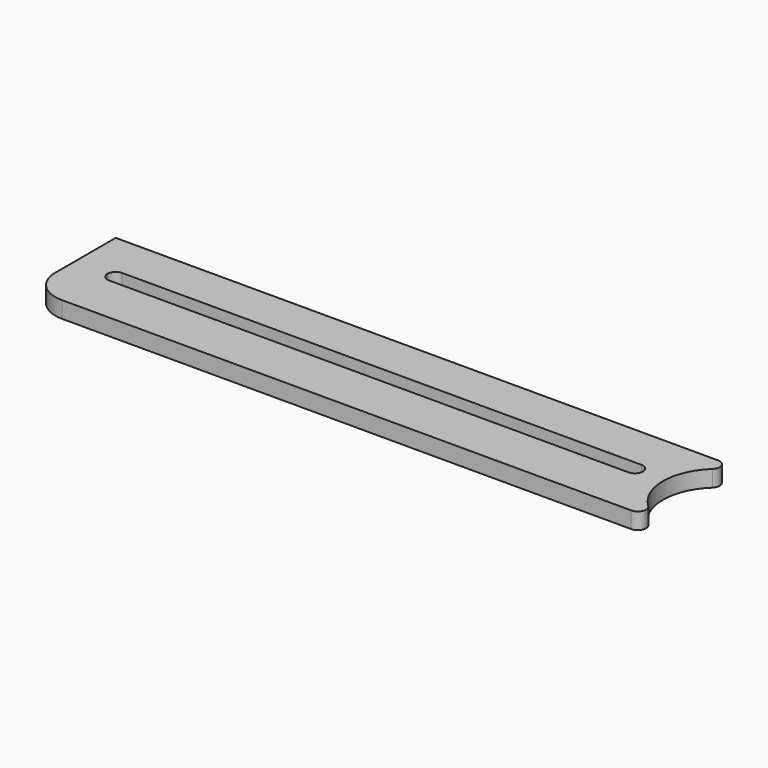
from build123d import *

# Parameters (mm, degrees)
F0_W         = 99.7252352536
F0_H         = 16.7486164719
F1_DEPTH     = 2.54
F2_R         = 5.08
F3_R         = 8.5048235264
F4_DEPTH     = 2.54
F5_W         = 82.7053110433
F5_H         = 2.5119255297
F6_DEPTH     = 2.54
F7_R         = 1.27
F8_T1_DEPTH  = 2.54
F9_R         = 1.27
F10_T1_DEPTH = 2.54
F11_R        = 1.27
F12_R        = 1.27


# Not quite as in the source:
# - a fillet or chamfer that OpenCascade refuses, or shapes differently, is made with other operations: its cross-section is extruded or revolved along the edge and cut away or added


with BuildPart() as f1:
    # F0 (on Top) → F1 (new body)
    with BuildSketch(Plane.XY):
        with Locations((-11.1071113497, -8.3743082359)):
            Rectangle(F0_W, F0_H)
    extrude(amount=F1_DEPTH)

    # F2
    f2_edges = [f1.edges().sort_by_distance(p)[0] for p in [
        (-60.969729, -16.748616, 1.27),
    ]]
    fillet(f2_edges, radius=F2_R)

    # F3 (on face) → F4 (cut)
    with BuildSketch(Plane.XY.offset(2.54)):
        with Locations((38.7555062771, -8.3743082359)):
            Circle(F3_R)
    extrude(amount=-F4_DEPTH, mode=Mode.SUBTRACT)

    # F5 (on face) → F6 (cut)
    with BuildSketch(Plane(origin=(0, 0, 0), x_dir=(1, 0, 0), z_dir=(0, 0, -1))):
        with Locations((-14.5370734549, 7.9348592553)):
            Rectangle(F5_W, F5_H)
    extrude(amount=-F6_DEPTH, mode=Mode.SUBTRACT)

    # F7
    f7_edges = [f1.edges().sort_by_distance(p)[0] for p in [
        (-55.889729, -9.190822, 1.27),
    ]]
    fillet(f7_edges, radius=F7_R)

    # F8: fillet of radius 1.27 on 1 edges, made by hand

    # F8_s2 → F8_t1 (join)
    with BuildSketch(Plane.XY):
        with BuildLine():
            ThreePointArc((-55.8897289765, -7.9488964905), (-55.5177545886, -7.0508708784), (-54.6197289765, -6.6788964905))
            Line((-54.6197289765, -6.6788964905), (-55.8897289765, -6.6788964905))
            Line((-55.8897289765, -6.6788964905), (-55.8897289765, -7.9488964905))
        make_face()
    extrude(amount=F8_T1_DEPTH)

    # F9
    f9_edges = [f1.edges().sort_by_distance(p)[0] for p in [
        (26.815582, -6.678896, 1.27),
    ]]
    fillet(f9_edges, radius=F9_R)

    # F10: fillet of radius 1.27 on 1 edges, made by hand

    # F10_s2 → F10_t1 (join)
    with BuildSketch(Plane.XY):
        with BuildLine():
            ThreePointArc((26.8155820668, -7.9208220202), (26.4436076789, -8.8188476323), (25.5455820668, -9.1908220202))
            Line((25.5455820668, -9.1908220202), (26.8155820668, -9.1908220202))
            Line((26.8155820668, -9.1908220202), (26.8155820668, -7.9208220202))
        make_face()
    extrude(amount=F10_T1_DEPTH)

    # F11
    f11_edges = [f1.edges().sort_by_distance(p)[0] for p in [
        (37.271261, -16.748616, 1.27),
    ]]
    fillet(f11_edges, radius=F11_R)

    # F12
    f12_edges = [f1.edges().sort_by_distance(p)[0] for p in [
        (37.271261, 0, 1.27),
    ]]
    fillet(f12_edges, radius=F12_R)


solid = f1.part
